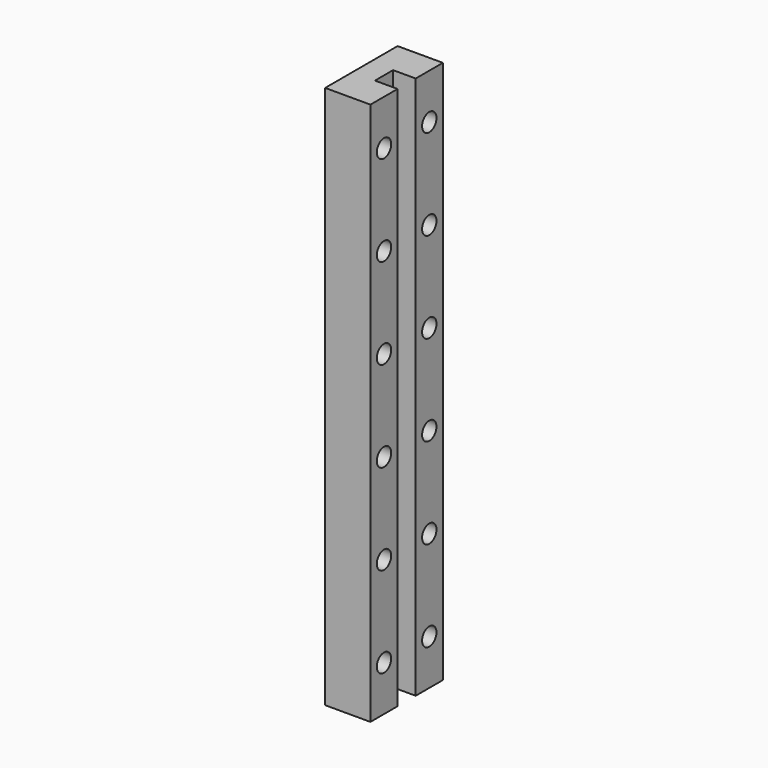
from build123d import *

# Parameters (mm, degrees)
F0_W      = 50.8
F0_H      = 304.8
F1_DEPTH  = 12.7
F3_W      = 12.7
F3_H      = 12.7
F4_DEPTH  = 304.8
F7_D      = 10.0838
F7_DEPTH  = 30.48
F7_TIP    = 3.0294791551
F9_R      = 7.54126
F9_R_2    = 3.302
F10_DEPTH = 6.35
F12_D     = 6.35
F12_DEPTH = 30.48
F12_TIP   = 1.9077324654
F13_R     = 5.0419
F13_R_2   = 2.54
F14_DEPTH = 7.62


# Not quite as in the source:
# - a feature names something its author has since deleted; it is built from what else it names


with BuildPart() as f1:
    # F0 (on Right) → F1 (new body, symmetric)
    with BuildSketch(Plane.YZ):
        Rectangle(F0_W, F0_H)
    extrude(amount=F1_DEPTH, both=True)

    # F3 (on offset) → F4 (cut)
    with BuildSketch(Plane.XY.offset(-152.4)):
        with Locations((6.35, 0)):
            Rectangle(F3_W, F3_H)
    extrude(amount=F4_DEPTH, mode=Mode.SUBTRACT)

    # F7
    with Locations(Plane.YZ.offset(12.7)):
        with Locations((-15.875, 76.2), (15.875, 76.2), (15.875, 25.4), (-15.875, 25.4), (-15.875, -25.4), (15.875, -25.4), (15.875, -127), (-15.875, -127), (-15.875, -76.2), (15.875, -76.2), (-15.875, 127), (15.875, 127)):
            Hole(F7_D / 2, depth=F7_DEPTH)
            with Locations((0, 0, -(F7_DEPTH + F7_TIP / 2))):  # 118° drill point
                Cone(0, F7_D / 2, F7_TIP, mode=Mode.SUBTRACT)

    # F9 (on offset) → F10 (cut)
    with BuildSketch(Plane.YZ.offset(-12.7)):
        with Locations((15.875, 127)):
            Circle(F9_R)
        with Locations((15.875, 127)):
            Circle(F9_R_2, mode=Mode.SUBTRACT)
        with Locations((-15.875, 127)):
            Circle(F9_R)
        with Locations((-15.875, 127)):
            Circle(F9_R_2, mode=Mode.SUBTRACT)
        with Locations((-15.875, 76.2)):
            Circle(F9_R)
        with Locations((-15.875, 76.2)):
            Circle(F9_R_2, mode=Mode.SUBTRACT)
        with Locations((15.875, 76.2)):
            Circle(F9_R)
        with Locations((15.875, 76.2)):
            Circle(F9_R_2, mode=Mode.SUBTRACT)
        with Locations((15.875, 25.4)):
            Circle(F9_R)
        with Locations((15.875, 25.4)):
            Circle(F9_R_2, mode=Mode.SUBTRACT)
        with Locations((-15.875, 25.4)):
            Circle(F9_R)
        with Locations((-15.875, 25.4)):
            Circle(F9_R_2, mode=Mode.SUBTRACT)
        with Locations((15.875, -25.4)):
            Circle(F9_R)
        with Locations((15.875, -25.4)):
            Circle(F9_R_2, mode=Mode.SUBTRACT)
        with Locations((-15.875, -25.4)):
            Circle(F9_R)
        with Locations((-15.875, -25.4)):
            Circle(F9_R_2, mode=Mode.SUBTRACT)
        with Locations((-15.875, -76.2)):
            Circle(F9_R)
        with Locations((-15.875, -76.2)):
            Circle(F9_R_2, mode=Mode.SUBTRACT)
        with Locations((15.875, -76.2)):
            Circle(F9_R)
        with Locations((15.875, -76.2)):
            Circle(F9_R_2, mode=Mode.SUBTRACT)
        with Locations((15.875, -127)):
            Circle(F9_R)
        with Locations((15.875, -127)):
            Circle(F9_R_2, mode=Mode.SUBTRACT)
        with Locations((-15.875, -127)):
            Circle(F9_R)
        with Locations((-15.875, -127)):
            Circle(F9_R_2, mode=Mode.SUBTRACT)
    extrude(amount=F10_DEPTH, mode=Mode.SUBTRACT)

    # F12
    with Locations(Plane(origin=(-12.7, 0, 0), x_dir=(0, 1, 0), z_dir=(-1, 0, 0))):
        with Locations((0, -139.7), (0, -114.3), (0, -88.9), (0, -63.5), (0, -38.1), (0, 12.7), (0, -12.7), (0, 38.1), (0, 63.5), (0, 114.3), (0, 139.7), (0, 88.9)):
            Hole(F12_D / 2, depth=F12_DEPTH)
            with Locations((0, 0, -(F12_DEPTH + F12_TIP / 2))):  # 118° drill point
                Cone(0, F12_D / 2, F12_TIP, mode=Mode.SUBTRACT)

    # F13 (on offset) → F14 (cut)
    with BuildSketch(Plane.YZ.offset(-12.7)):
        with Locations((0, 139.7)):
            Circle(F13_R)
        with Locations((0, 139.7)):
            Circle(F13_R_2, mode=Mode.SUBTRACT)
        with Locations((0, 114.3)):
            Circle(F13_R)
        with Locations((0, 114.3)):
            Circle(F13_R_2, mode=Mode.SUBTRACT)
        with Locations((0, 88.9)):
            Circle(F13_R)
        with Locations((0, 88.9)):
            Circle(F13_R_2, mode=Mode.SUBTRACT)
        with Locations((0, 63.5)):
            Circle(F13_R)
        with Locations((0, 63.5)):
            Circle(F13_R_2, mode=Mode.SUBTRACT)
        with Locations((0, 38.1)):
            Circle(F13_R)
        with Locations((0, 38.1)):
            Circle(F13_R_2, mode=Mode.SUBTRACT)
        with Locations((0, 12.7)):
            Circle(F13_R)
        with Locations((0, 12.7)):
            Circle(F13_R_2, mode=Mode.SUBTRACT)
        with Locations((0, -12.7)):
            Circle(F13_R)
        with Locations((0, -12.7)):
            Circle(F13_R_2, mode=Mode.SUBTRACT)
        with Locations((0, -38.1)):
            Circle(F13_R)
        with Locations((0, -38.1)):
            Circle(F13_R_2, mode=Mode.SUBTRACT)
        with Locations((0, -63.5)):
            Circle(F13_R)
        with Locations((0, -63.5)):
            Circle(F13_R_2, mode=Mode.SUBTRACT)
        with Locations((0, -88.9)):
            Circle(F13_R)
        with Locations((0, -88.9)):
            Circle(F13_R_2, mode=Mode.SUBTRACT)
        with Locations((0, -114.3)):
            Circle(F13_R)
        with Locations((0, -114.3)):
            Circle(F13_R_2, mode=Mode.SUBTRACT)
        with Locations((0, -139.7)):
            Circle(F13_R)
        with Locations((0, -139.7)):
            Circle(F13_R_2, mode=Mode.SUBTRACT)
    extrude(amount=F14_DEPTH, mode=Mode.SUBTRACT)


solid = f1.part
